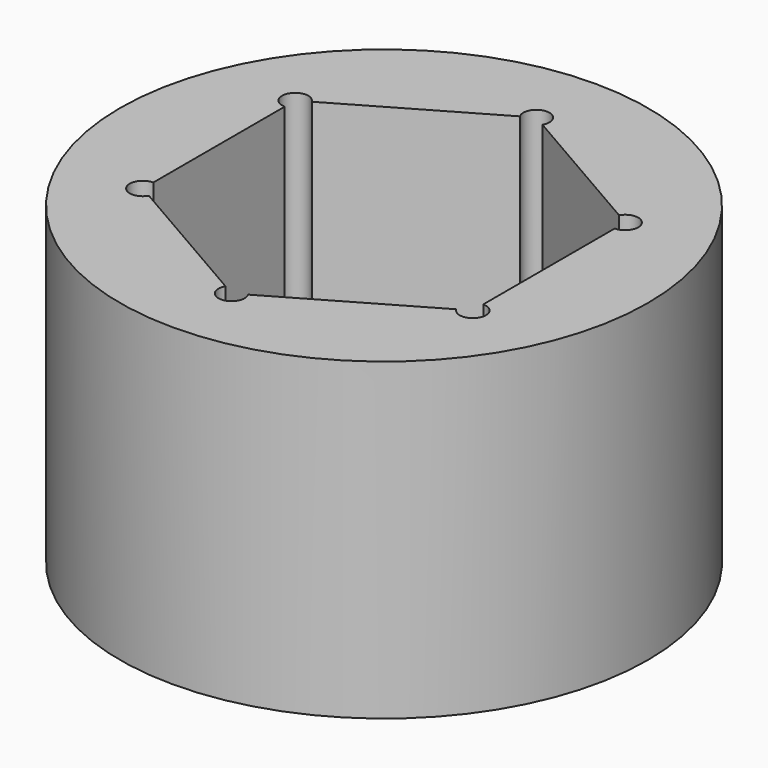
from build123d import *

# Parameters (mm, degrees)
F0_R     = 8
F1_DEPTH = 9.525


# Not quite as in the source:
# - a length typed as a fraction of an inch, garbled in the dataset ("3 / 203.2 mm" for 3/8 in), is restored


with BuildPart() as f1:
    # F0 (on Top) → F1 (new body)
    with BuildSketch(Plane.XY):
        Circle(F0_R)
        with BuildLine():
            ThreePointArc((-0.3437038321, 5.5750625), (0, 6.170375), (0.3437038321, 5.5750625))
            Line((0.3437038321, 5.5750625), (4.6562938366, 3.0851875))
            ThreePointArc((4.6562938366, 3.0851875), (5.3437015009, 3.0851875), (4.9999976687, 2.489875))
            Line((4.9999976687, 2.489875), (4.9999976687, -2.489875))
            ThreePointArc((4.9999976687, -2.489875), (5.3437015009, -3.0851875), (4.6562938366, -3.0851875))
            Line((4.6562938366, -3.0851875), (0.3437038321, -5.5750625))
            ThreePointArc((0.3437038321, -5.5750625), (0, -6.170375), (-0.3437038321, -5.5750625))
            Line((-0.3437038321, -5.5750625), (-4.6562938366, -3.0851875))
            ThreePointArc((-4.6562938366, -3.0851875), (-5.3437015009, -3.0851875), (-4.9999976687, -2.489875))
            Line((-4.9999976687, -2.489875), (-4.9999976687, 2.489875))
            ThreePointArc((-4.9999976687, 2.489875), (-5.3437015009, 3.0851875), (-4.6562938366, 3.0851875))
            Line((-4.6562938366, 3.0851875), (-0.3437038321, 5.5750625))
        make_face(mode=Mode.SUBTRACT)
    extrude(amount=F1_DEPTH)


solid = f1.part
